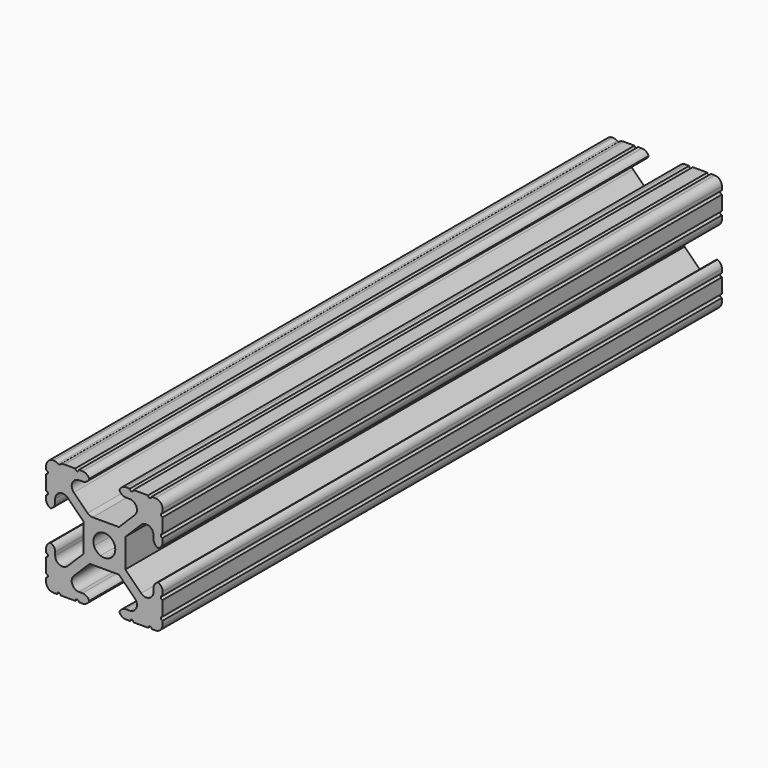
from build123d import *

# Parameters (mm, degrees)
F1_DEPTH    = 152.4
F2_T1_DEPTH = 152.4
F2_T3_DEPTH = 160.3375
F2_T5_DEPTH = 156.36875


# Not quite as in the source:
# - a fillet or chamfer that OpenCascade refuses, or shapes differently, is made with other operations: its cross-section is extruded or revolved along the edge and cut away or added


with BuildPart() as f1:
    # F0 (on Front) → F1 (new body)
    with BuildSketch(Plane.XZ):
        with BuildLine():
            ThreePointArc((-0.8361427067, 2.2296225996), (0, 2.38125), (0.8361427067, 2.2296225996))
            Line((0.8361427067, 2.2296225996), (3.1853789104, 4.5640625))
            Line((3.1853789104, 4.5640625), (-3.1853789104, 4.5640625))
            Line((-3.1853789104, 4.5640625), (-0.8361427067, 2.2296225996))
        make_face()
        with BuildLine():
            ThreePointArc((-2.2347427098, 0.8223603732), (-1.6889881746, 1.6785918231), (-0.8361427067, 2.2296225996))
            Line((-0.8361427067, 2.2296225996), (-3.1853789104, 4.5640625))
            Line((-3.1853789104, 4.5640625), (-4.5640625, 4.5640625))
            Line((-4.5640625, 4.5640625), (-4.5640625, 3.1376763557))
            Line((-4.5640625, 3.1376763557), (-2.2347427098, 0.8223603732))
        make_face()
        with BuildLine():
            ThreePointArc((-2.2347427098, -0.8223603732), (-2.38125, 0), (-2.2347427098, 0.8223603732))
            Line((-2.2347427098, 0.8223603732), (-4.5640625, 3.1376763557))
            Line((-4.5640625, 3.1376763557), (-4.5640625, -3.1376763557))
            Line((-4.5640625, -3.1376763557), (-2.2347427098, -0.8223603732))
        make_face()
        with BuildLine():
            Line((-3.1853789104, -4.5640625), (-0.8361427067, -2.2296225996))
            ThreePointArc((-0.8361427067, -2.2296225996), (-1.6889881746, -1.6785918231), (-2.2347427098, -0.8223603732))
            Line((-2.2347427098, -0.8223603732), (-4.5640625, -3.1376763557))
            Line((-4.5640625, -3.1376763557), (-4.5640625, -4.5640625))
            Line((-4.5640625, -4.5640625), (-3.1853789104, -4.5640625))
        make_face()
        with BuildLine():
            Line((3.1853789104, -4.5640625), (0.8361427067, -2.2296225996))
            ThreePointArc((0.8361427067, -2.2296225996), (0, -2.38125), (-0.8361427067, -2.2296225996))
            Line((-0.8361427067, -2.2296225996), (-3.1853789104, -4.5640625))
            Line((-3.1853789104, -4.5640625), (3.1853789104, -4.5640625))
        make_face()
        with BuildLine():
            Line((4.5640625, -3.1376763557), (2.2347427098, -0.8223603732))
            ThreePointArc((2.2347427098, -0.8223603732), (1.6889881746, -1.6785918231), (0.8361427067, -2.2296225996))
            Line((0.8361427067, -2.2296225996), (3.1853789104, -4.5640625))
            Line((3.1853789104, -4.5640625), (4.5640625, -4.5640625))
            Line((4.5640625, -4.5640625), (4.5640625, -3.1376763557))
        make_face()
        with BuildLine():
            ThreePointArc((2.2347427098, 0.8223603732), (2.3443370748, 0.4176544533), (2.38125, 0))
            ThreePointArc((2.38125, 0), (2.3443370748, -0.4176544533), (2.2347427098, -0.8223603732))
            Line((2.2347427098, -0.8223603732), (4.5640625, -3.1376763557))
            Line((4.5640625, -3.1376763557), (4.5640625, 3.1376763557))
            Line((4.5640625, 3.1376763557), (2.2347427098, 0.8223603732))
        make_face()
        with BuildLine():
            ThreePointArc((0.8361427067, 2.2296225996), (1.6889881746, 1.6785918231), (2.2347427098, 0.8223603732))
            Line((2.2347427098, 0.8223603732), (4.5640625, 3.1376763557))
            Line((4.5640625, 3.1376763557), (4.5640625, 4.5640625))
            Line((4.5640625, 4.5640625), (3.1853789104, 4.5640625))
            Line((3.1853789104, 4.5640625), (0.8361427067, 2.2296225996))
        make_face()
        Polygon((4.5640625, 4.5640625), (4.5640625, 3.1376763557), (10.715625, 9.2522558281), (12.7, 11.2247008192), (12.7, 12.7), (11.3728841543, 12.7), (9.3759316558, 10.715625), (3.1853789104, 4.5640625), align=None)
        with BuildLine():
            Line((12.7, 11.2247008192), (10.715625, 9.2522558281))
            Line((10.715625, 9.2522558281), (10.715625, 7.14375))
            Line((10.715625, 7.14375), (10.715625, 3.175))
            Line((10.715625, 3.175), (12.7, 3.175))
            Line((12.7, 3.175), (12.7, 5.55625))
            ThreePointArc((12.7, 5.55625), (12.303125, 5.953125), (12.7, 6.35))
            Line((12.7, 6.35), (12.7, 9.525))
            ThreePointArc((12.7, 9.525), (12.303125, 9.921875), (12.7, 10.31875))
            Line((12.7, 10.31875), (12.7, 11.2247008192))
        make_face()
        with BuildLine():
            Line((7.14375, 10.715625), (9.3759316558, 10.715625))
            Line((9.3759316558, 10.715625), (11.3728841543, 12.7))
            Line((11.3728841543, 12.7), (10.31875, 12.7))
            ThreePointArc((10.31875, 12.7), (9.921875, 12.303125), (9.525, 12.7))
            Line((9.525, 12.7), (6.35, 12.7))
            ThreePointArc((6.35, 12.7), (5.953125, 12.303125), (5.55625, 12.7))
            Line((5.55625, 12.7), (3.175, 12.7))
            Line((3.175, 12.7), (3.175, 10.715625))
            Line((3.175, 10.715625), (7.14375, 10.715625))
        make_face()
        with BuildLine():
            Line((-11.3728841543, 12.7), (-9.3759316558, 10.715625))
            Line((-9.3759316558, 10.715625), (-7.14375, 10.715625))
            Line((-7.14375, 10.715625), (-3.175, 10.715625))
            Line((-3.175, 10.715625), (-3.175, 12.7))
            Line((-3.175, 12.7), (-5.55625, 12.7))
            ThreePointArc((-5.55625, 12.7), (-5.953125, 12.303125), (-6.35, 12.7))
            Line((-6.35, 12.7), (-7.14375, 12.7))
            Line((-7.14375, 12.7), (-9.525, 12.7))
            ThreePointArc((-9.525, 12.7), (-9.921875, 12.303125), (-10.31875, 12.7))
            Line((-10.31875, 12.7), (-11.3728841543, 12.7))
        make_face()
        Polygon((-4.5640625, 4.5640625), (-3.1853789104, 4.5640625), (-9.3759316558, 10.715625), (-11.3728841543, 12.7), (-12.7, 11.2247008192), (-10.715625, 9.2522558281), (-4.5640625, 3.1376763557), align=None)
        Polygon((-12.7, 11.2247008192), (-11.3728841543, 12.7), (-12.7, 12.7), align=None)
        with BuildLine():
            Line((-10.715625, 7.14375), (-10.715625, 9.2522558281))
            Line((-10.715625, 9.2522558281), (-12.7, 11.2247008192))
            Line((-12.7, 11.2247008192), (-12.7, 10.31875))
            ThreePointArc((-12.7, 10.31875), (-12.303125, 9.921875), (-12.7, 9.525))
            Line((-12.7, 9.525), (-12.7, 6.35))
            ThreePointArc((-12.7, 6.35), (-12.303125, 5.953125), (-12.7, 5.55625))
            Line((-12.7, 5.55625), (-12.7, 3.175))
            Line((-12.7, 3.175), (-10.715625, 3.175))
            Line((-10.715625, 3.175), (-10.715625, 7.14375))
        make_face()
        with BuildLine():
            Line((-12.7, -11.2247008192), (-10.715625, -9.2522558281))
            Line((-10.715625, -9.2522558281), (-10.715625, -7.14375))
            Line((-10.715625, -7.14375), (-10.715625, -3.175))
            Line((-10.715625, -3.175), (-12.7, -3.175))
            Line((-12.7, -3.175), (-12.7, -5.55625))
            ThreePointArc((-12.7, -5.55625), (-12.303125, -5.953125), (-12.7, -6.35))
            Line((-12.7, -6.35), (-12.7, -9.525))
            ThreePointArc((-12.7, -9.525), (-12.303125, -9.921875), (-12.7, -10.31875))
            Line((-12.7, -10.31875), (-12.7, -11.2247008192))
        make_face()
        Polygon((-9.3759316558, -10.715625), (-3.1853789104, -4.5640625), (-4.5640625, -4.5640625), (-4.5640625, -3.1376763557), (-10.715625, -9.2522558281), (-12.7, -11.2247008192), (-12.7, -12.7), (-11.3728841543, -12.7), align=None)
        with BuildLine():
            Line((-7.14375, -10.715625), (-9.3759316558, -10.715625))
            Line((-9.3759316558, -10.715625), (-11.3728841543, -12.7))
            Line((-11.3728841543, -12.7), (-10.31875, -12.7))
            ThreePointArc((-10.31875, -12.7), (-9.921875, -12.303125), (-9.525, -12.7))
            Line((-9.525, -12.7), (-6.35, -12.7))
            ThreePointArc((-6.35, -12.7), (-5.953125, -12.303125), (-5.55625, -12.7))
            Line((-5.55625, -12.7), (-3.175, -12.7))
            Line((-3.175, -12.7), (-3.175, -10.715625))
            Line((-3.175, -10.715625), (-7.14375, -10.715625))
        make_face()
        with BuildLine():
            Line((11.3728841543, -12.7), (9.3759316558, -10.715625))
            Line((9.3759316558, -10.715625), (7.14375, -10.715625))
            Line((7.14375, -10.715625), (3.175, -10.715625))
            Line((3.175, -10.715625), (3.175, -12.7))
            Line((3.175, -12.7), (5.55625, -12.7))
            ThreePointArc((5.55625, -12.7), (5.953125, -12.303125), (6.35, -12.7))
            Line((6.35, -12.7), (9.525, -12.7))
            ThreePointArc((9.525, -12.7), (9.921875, -12.303125), (10.31875, -12.7))
            Line((10.31875, -12.7), (11.3728841543, -12.7))
        make_face()
        Polygon((10.715625, -9.2522558281), (4.5640625, -3.1376763557), (4.5640625, -4.5640625), (3.1853789104, -4.5640625), (9.3759316558, -10.715625), (11.3728841543, -12.7), (12.7, -12.7), (12.7, -11.2247008192), align=None)
        with BuildLine():
            Line((10.715625, -7.14375), (10.715625, -9.2522558281))
            Line((10.715625, -9.2522558281), (12.7, -11.2247008192))
            Line((12.7, -11.2247008192), (12.7, -10.31875))
            ThreePointArc((12.7, -10.31875), (12.303125, -9.921875), (12.7, -9.525))
            Line((12.7, -9.525), (12.7, -6.35))
            ThreePointArc((12.7, -6.35), (12.303125, -5.953125), (12.7, -5.55625))
            Line((12.7, -5.55625), (12.7, -3.175))
            Line((12.7, -3.175), (10.715625, -3.175))
            Line((10.715625, -3.175), (10.715625, -7.14375))
        make_face()
    extrude(amount=F1_DEPTH)

    # F2: fillet of radius 1.5875 on 31 edges, made by hand

    # F2_s2 → F2_t1 (join)
    with BuildSketch(Plane.XZ):
        with BuildLine():
            ThreePointArc((-6.6451596968, 8.0020523886), (-6.9937960043, 9.7333175229), (-5.5261794807, 10.715625))
            Line((-5.5261794807, 10.715625), (-9.3759316558, 10.715625))
            Line((-9.3759316558, 10.715625), (-6.6451596968, 8.0020523886))
        make_face()
        with BuildLine():
            ThreePointArc((-8.0089825615, 6.5618856508), (-9.7378452755, 6.9017155215), (-10.715625, 5.4359742634))
            Line((-10.715625, 5.4359742634), (-10.715625, 9.2522558281))
            Line((-10.715625, 9.2522558281), (-8.0089825615, 6.5618856508))
        make_face()
        with BuildLine():
            ThreePointArc((5.5261794807, 10.715625), (6.9937960043, 9.7333175229), (6.6451596968, 8.0020523886))
            Line((6.6451596968, 8.0020523886), (9.3759316558, 10.715625))
            Line((9.3759316558, 10.715625), (5.5261794807, 10.715625))
        make_face()
        with BuildLine():
            ThreePointArc((8.0089825615, 6.5618856508), (9.7378452755, 6.9017155215), (10.715625, 5.4359742634))
            Line((10.715625, 5.4359742634), (10.715625, 9.2522558281))
            Line((10.715625, 9.2522558281), (8.0089825615, 6.5618856508))
        make_face()
        with BuildLine():
            ThreePointArc((10.715625, -5.4359742634), (9.7378452755, -6.9017155215), (8.0089825615, -6.5618856508))
            Line((8.0089825615, -6.5618856508), (10.715625, -9.2522558281))
            Line((10.715625, -9.2522558281), (10.715625, -5.4359742634))
        make_face()
        with BuildLine():
            ThreePointArc((6.6451596968, -8.0020523886), (6.9937960043, -9.7333175229), (5.5261794807, -10.715625))
            Line((5.5261794807, -10.715625), (9.3759316558, -10.715625))
            Line((9.3759316558, -10.715625), (6.6451596968, -8.0020523886))
        make_face()
        with BuildLine():
            ThreePointArc((-5.5261794807, -10.715625), (-6.9937960043, -9.7333175229), (-6.6451596968, -8.0020523886))
            Line((-6.6451596968, -8.0020523886), (-9.3759316558, -10.715625))
            Line((-9.3759316558, -10.715625), (-5.5261794807, -10.715625))
        make_face()
        with BuildLine():
            ThreePointArc((-8.0089825615, -6.5618856508), (-9.7378452755, -6.9017155215), (-10.715625, -5.4359742634))
            Line((-10.715625, -5.4359742634), (-10.715625, -9.2522558281))
            Line((-10.715625, -9.2522558281), (-8.0089825615, -6.5618856508))
        make_face()
        with BuildLine():
            ThreePointArc((-2.530750733, 4.5640625), (-3.1359432558, 4.6839459764), (-3.649730949, 5.0254898886))
            Line((-3.649730949, 5.0254898886), (-3.1853789104, 4.5640625))
            Line((-3.1853789104, 4.5640625), (-2.530750733, 4.5640625))
        make_face()
    extrude(amount=F2_T1_DEPTH)

    # F2_s4 → F2_t3 (cut)
    with BuildSketch(Plane.XZ.offset(-3.96875)):
        with BuildLine():
            ThreePointArc((-12.7, -11.1125), (-12.2350320151, -12.2350320151), (-11.1125, -12.7))
            Line((-11.1125, -12.7), (-12.7, -12.7))
            Line((-12.7, -12.7), (-12.7, -11.1125))
        make_face()
        with BuildLine():
            ThreePointArc((11.1125, -12.7), (12.2350320151, -12.2350320151), (12.7, -11.1125))
            Line((12.7, -11.1125), (12.7, -12.7))
            Line((12.7, -12.7), (11.1125, -12.7))
        make_face()
        with BuildLine():
            ThreePointArc((12.7, 11.1125), (12.2350320151, 12.2350320151), (11.1125, 12.7))
            Line((11.1125, 12.7), (12.7, 12.7))
            Line((12.7, 12.7), (12.7, 11.1125))
        make_face()
        with BuildLine():
            ThreePointArc((-12.7, 4.7625), (-12.2350320151, 3.6399679849), (-11.1125, 3.175))
            Line((-11.1125, 3.175), (-12.7, 3.175))
            Line((-12.7, 3.175), (-12.7, 4.7625))
        make_face()
        with BuildLine():
            ThreePointArc((-11.1125, -3.175), (-12.2350320151, -3.6399679849), (-12.7, -4.7625))
            Line((-12.7, -4.7625), (-12.7, -3.175))
            Line((-12.7, -3.175), (-11.1125, -3.175))
        make_face()
        with BuildLine():
            ThreePointArc((-12.303125, 3.175), (-11.1805929849, 3.6399679849), (-10.715625, 4.7625))
            Line((-10.715625, 4.7625), (-10.715625, 3.175))
            Line((-10.715625, 3.175), (-12.303125, 3.175))
        make_face()
        with BuildLine():
            ThreePointArc((-10.715625, -4.7625), (-11.1805929849, -3.6399679849), (-12.303125, -3.175))
            Line((-12.303125, -3.175), (-10.715625, -3.175))
            Line((-10.715625, -3.175), (-10.715625, -4.7625))
        make_face()
        with BuildLine():
            ThreePointArc((-3.175, -12.303125), (-3.6399679849, -11.1805929849), (-4.7625, -10.715625))
            Line((-4.7625, -10.715625), (-3.175, -10.715625))
            Line((-3.175, -10.715625), (-3.175, -12.303125))
        make_face()
        with BuildLine():
            ThreePointArc((-4.7625, -12.7), (-3.6399679849, -12.2350320151), (-3.175, -11.1125))
            Line((-3.175, -11.1125), (-3.175, -12.7))
            Line((-3.175, -12.7), (-4.7625, -12.7))
        make_face()
        with BuildLine():
            ThreePointArc((3.175, -11.1125), (3.6399679849, -12.2350320151), (4.7625, -12.7))
            Line((4.7625, -12.7), (3.175, -12.7))
            Line((3.175, -12.7), (3.175, -11.1125))
        make_face()
        with BuildLine():
            ThreePointArc((4.7625, -10.715625), (3.6399679849, -11.1805929849), (3.175, -12.303125))
            Line((3.175, -12.303125), (3.175, -10.715625))
            Line((3.175, -10.715625), (4.7625, -10.715625))
        make_face()
        with BuildLine():
            ThreePointArc((12.7, -4.7625), (12.2350320151, -3.6399679849), (11.1125, -3.175))
            Line((11.1125, -3.175), (12.7, -3.175))
            Line((12.7, -3.175), (12.7, -4.7625))
        make_face()
        with BuildLine():
            ThreePointArc((11.1125, 3.175), (12.2350320151, 3.6399679849), (12.7, 4.7625))
            Line((12.7, 4.7625), (12.7, 3.175))
            Line((12.7, 3.175), (11.1125, 3.175))
        make_face()
        with BuildLine():
            ThreePointArc((12.303125, -3.175), (11.1805929849, -3.6399679849), (10.715625, -4.7625))
            Line((10.715625, -4.7625), (10.715625, -3.175))
            Line((10.715625, -3.175), (12.303125, -3.175))
        make_face()
        with BuildLine():
            ThreePointArc((10.715625, 4.7625), (11.1805929849, 3.6399679849), (12.303125, 3.175))
            Line((12.303125, 3.175), (10.715625, 3.175))
            Line((10.715625, 3.175), (10.715625, 4.7625))
        make_face()
        with BuildLine():
            ThreePointArc((-4.7625, 10.715625), (-3.6399679849, 11.1805929849), (-3.175, 12.303125))
            Line((-3.175, 12.303125), (-3.175, 10.715625))
            Line((-3.175, 10.715625), (-4.7625, 10.715625))
        make_face()
        with BuildLine():
            ThreePointArc((-3.175, 11.1125), (-3.6399679849, 12.2350320151), (-4.7625, 12.7))
            Line((-4.7625, 12.7), (-3.175, 12.7))
            Line((-3.175, 12.7), (-3.175, 11.1125))
        make_face()
        with BuildLine():
            ThreePointArc((4.7625, 12.7), (3.6399679849, 12.2350320151), (3.175, 11.1125))
            Line((3.175, 11.1125), (3.175, 12.7))
            Line((3.175, 12.7), (4.7625, 12.7))
        make_face()
        with BuildLine():
            ThreePointArc((3.175, 12.303125), (3.6399679849, 11.1805929849), (4.7625, 10.715625))
            Line((4.7625, 10.715625), (3.175, 10.715625))
            Line((3.175, 10.715625), (3.175, 12.303125))
        make_face()
        with BuildLine():
            ThreePointArc((-11.1125, 12.7), (-12.2350320151, 12.2350320151), (-12.7, 11.1125))
            Line((-12.7, 11.1125), (-12.7, 12.7))
            Line((-12.7, 12.7), (-11.1125, 12.7))
        make_face()
    extrude(amount=F2_T3_DEPTH, mode=Mode.SUBTRACT)

    # F2_s6 → F2_t5 (cut)
    with BuildSketch(Plane.XZ.offset(-1.984375)):
        with BuildLine():
            ThreePointArc((-8.73125, 12.7), (-9.2332615786, 12.6185347357), (-9.68375, 12.3825))
            ThreePointArc((-9.68375, 12.3825), (-9.5668992086, 12.5225121043), (-9.525, 12.7))
            Line((-9.525, 12.7), (-8.73125, 12.7))
        make_face()
        with BuildLine():
            ThreePointArc((-10.16, 12.3825), (-10.6104884214, 12.6185347357), (-11.1125, 12.7))
            Line((-11.1125, 12.7), (-10.31875, 12.7))
            ThreePointArc((-10.31875, 12.7), (-10.2768507914, 12.5225121043), (-10.16, 12.3825))
        make_face()
    extrude(amount=F2_T5_DEPTH, mode=Mode.SUBTRACT)


solid = f1.part
